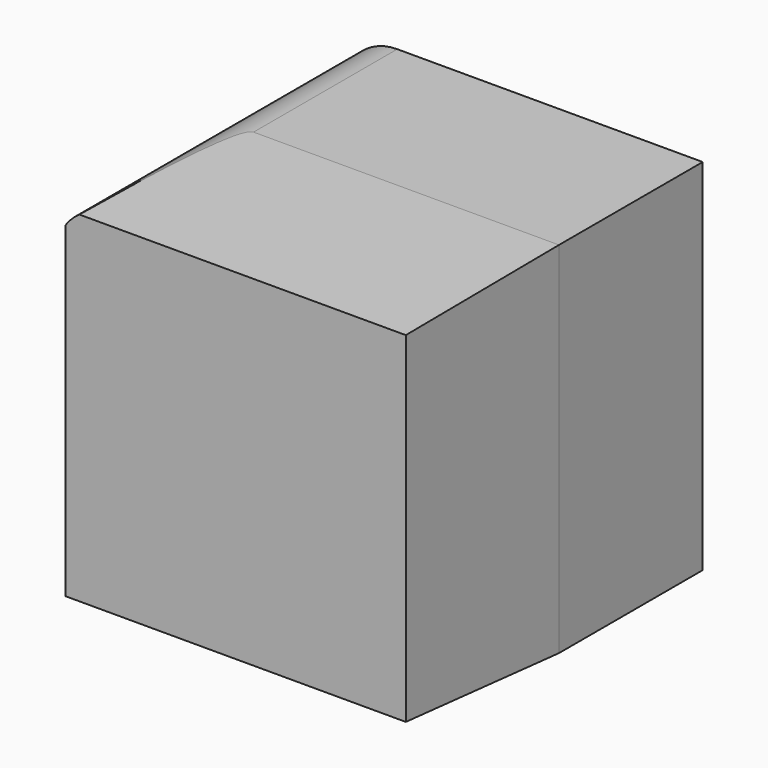
from build123d import *

# Parameters (mm, degrees)
F0_W          = 50.8
F0_H          = 50.8
F1_DEPTH      = 25.4
F1_TAPER      = 3
F1_DEPTH_BACK = 25.4
F2_T1_DEPTH   = 116.84


# Not quite as in the source:
# - a fillet or chamfer that OpenCascade refuses, or shapes differently, is made with other operations: its cross-section is extruded or revolved along the edge and cut away or added


with BuildPart() as f1:
    # F0 (on Front) → F1 (new body, two sides)
    with BuildSketch(Plane.XZ) as f1_sk:
        Rectangle(F0_W, F0_H)
    extrude(amount=F1_DEPTH, taper=F1_TAPER)
    extrude(f1_sk.sketch, amount=-F1_DEPTH_BACK)

    # F2: fillet of radius 7.62 on 1 edges, made by hand

    # F2_s2 → F2_t1 (cut)
    with BuildSketch(Plane.XZ.offset(-71.12)):
        with BuildLine():
            ThreePointArc((-25.4, 17.78), (-23.1681536726, 23.1681536726), (-17.78, 25.4))
            Line((-17.78, 25.4), (-17.78, 25.5524))
            Line((-17.78, 25.5524), (-25.5524, 25.5524))
            Line((-25.5524, 25.5524), (-25.5524, 17.78))
            Line((-25.5524, 17.78), (-25.4, 17.78))
        make_face()
    extrude(amount=F2_T1_DEPTH, mode=Mode.SUBTRACT)


solid = f1.part
